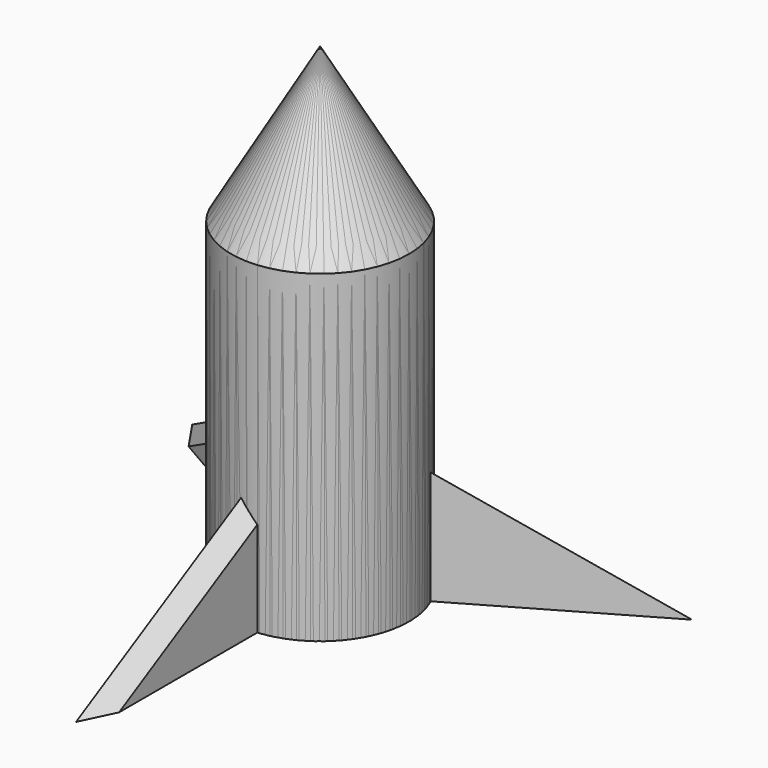
from build123d import *

# Parameters (mm, degrees)
F0_R        = 13.97
F0_R_2      = 11.43
F1_DEPTH    = 50.8
F2_R        = 13.97
F3_DEPTH    = 25.4
F3_TAPER    = 30
F4_T        = 2.54
F6_DEPTH    = 1.27
F7_T4_DEPTH = 69.1194463987
F7_S5_R     = 13.97
F7_T6_DEPTH = 38
F8_COUNT    = 3


# Not quite as in the source:
# - a fillet or chamfer that OpenCascade refuses, or shapes differently, is made with other operations: its cross-section is extruded or revolved along the edge and cut away or added
# - a shell that OpenCascade refuses in one call is made with other operations: the cavity is built on its own and cut out


with BuildPart() as f1:
    # F0 (on Top) → F1 (new body)
    with BuildSketch(Plane.XY):
        Circle(F0_R)
        Circle(F0_R_2, mode=Mode.SUBTRACT)
    extrude(amount=F1_DEPTH)

    # F2 (on face) → F3 (join)
    with BuildSketch(Plane.XY.offset(50.8)):
        Circle(F2_R)
    extrude(amount=F3_DEPTH, taper=F3_TAPER)

    # F4: shell of thickness 2.54, made by hand


with BuildPart() as f4_core1:
    # F4_t2: copy of F1
    add(f1.part)

    # the walls: a layer under each face that stays
    f4_faces = [f4_core1.faces().sort_by_distance(p)[0] for p in [
        (-13.97, 0, 25.4),
        (-9.3133333333, -9.3133333333, 0),
        (-6.985, 0, 62.8983748909),
        (-11.43, 0, 25.4),
    ]]
    thicken(f4_faces, amount=-F4_T, mode=Mode.SUBTRACT)


with BuildPart() as f1_1:
    add(f1.part)

    # what is left inside the walls is the cavity
    f4_cavity = [f4_core1.part.solids().sort_by_distance(p)[0] for p in [
        (-7.336043, 0, 57.15955),
    ]]
    add(f4_cavity, mode=Mode.SUBTRACT)

    # F5 (on Right) → F6 (join, symmetric)
    with BuildSketch(Plane.YZ):
        Polygon((-51.5810400248, 0), (-12.6313772053, 0), (-12.6313772053, 21.4238818735), align=None)
    extrude(amount=F6_DEPTH, both=True)

    # F7: chamfer of 5.08 on 1 edges, made by hand


with BuildPart() as f7_tool2:
    # F7_s3 → F7_t4 (new body)
    with BuildSketch(Plane(origin=(0, 9.5154878212, 5.233901202), x_dir=(1, 0, 0), z_dir=(0, -0.87620102, -0.4819458191))):
        Polygon((-3.81, 24.8592665835), (1.27, 19.7792665835), (1.27, 24.8592665835), align=None)
    extrude(amount=F7_T4_DEPTH)

    # F7_s5 → F7_t6 (cut, symmetric)
    with BuildSketch(Plane.XY.offset(8.1)):
        Circle(F7_S5_R)
    extrude(amount=F7_T6_DEPTH, both=True, mode=Mode.SUBTRACT)


with BuildPart() as f1_2:
    add(f1_1.part)

    # F7_t1: cut F7_tool2
    add(f7_tool2.part, mode=Mode.SUBTRACT)


with BuildPart() as f8_1:
    # F8: instance of F1
    add(f1_2.part.rotate(Axis((0, 0, 0), (0, 0, 1)), 1 * 360 / F8_COUNT))


with BuildPart() as f8_2:
    # F8: instance of F1
    add(f1_2.part.rotate(Axis((0, 0, 0), (0, 0, 1)), 2 * 360 / F8_COUNT))


solid = Compound([f1_2.part, f8_1.part, f8_2.part])
